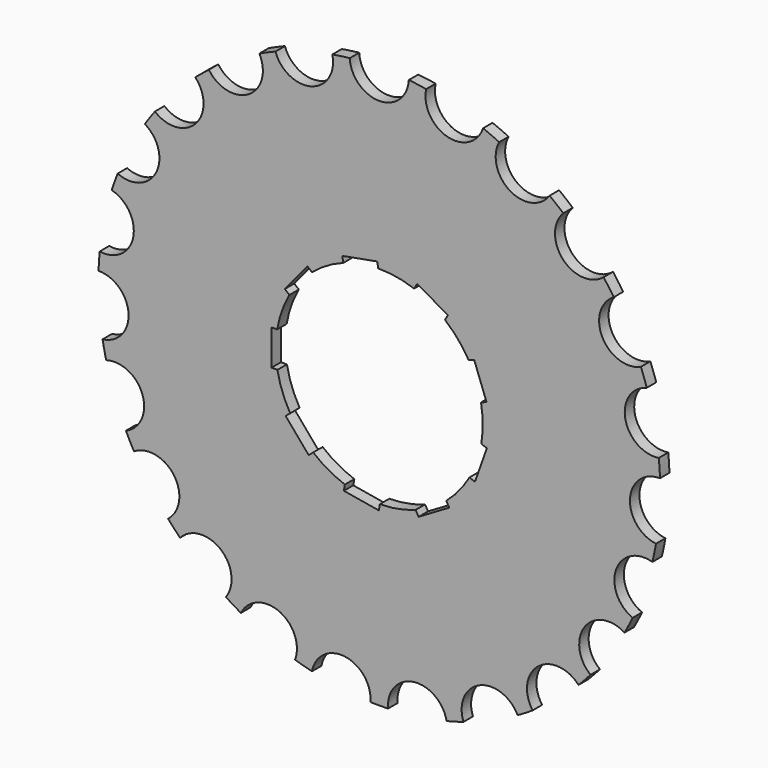
from build123d import *

# Parameters (mm, degrees)
F0_R            = 47.5
F0_R_2          = 17.5
F1_DEPTH        = 2
F3_DEPTH        = 2.001
F3_COPIES_COUNT = 23
F6_DEPTH        = 25
F6_COPIES_COUNT = 9


# Not quite as in the source:
# - a pattern or mirror of a feature is missing from the dataset's text; its kind, count and spacing are read off the source's solid


with BuildPart() as f1:
    # F0 (on Front) → F1 (new body)
    with BuildSketch(Plane.XZ):
        Circle(F0_R)
        Circle(F0_R_2, mode=Mode.SUBTRACT)
    extrude(amount=F1_DEPTH)

    # F2 (on face) → F3 (cut, through all)
    with BuildSketch(Plane.XZ.offset(2)):
        with BuildLine():
            ThreePointArc((4.9930699897, 47.2368421053), (0, 47.5), (-4.9930699897, 47.2368421053))
            ThreePointArc((-4.9930699897, 47.2368421053), (0, 42.5), (4.9930699897, 47.2368421053))
        make_face()
    f3 = extrude(amount=-F3_DEPTH, mode=Mode.SUBTRACT)

    # F3_copies: F3 ×23 about axis
    f3_copies_axis = Axis((0, 0, 0), (0, 1, 0))
    for i in range(1, F3_COPIES_COUNT):
        add(f3.rotate(f3_copies_axis, i * 360 / F3_COPIES_COUNT), mode=Mode.SUBTRACT)

    # F5 (on face) → F6 (cut)
    with BuildSketch(Plane.XZ.offset(2)):
        with BuildLine():
            Line((-6.2547624065, 17.3956841353), (-6.0736095937, 16.4122291753))
            ThreePointArc((-6.0736095937, 16.4122291753), (-3.1701742248, 17.2104618004), (-0.1728798335, 17.4991460524))
            Line((-0.1728798335, 17.4991460524), (-0.3540326464, 18.4826010124))
            Line((-0.3540326464, 18.4826010124), (-6.2547624065, 17.3956841353))
        make_face()
    f6 = extrude(amount=-F6_DEPTH, mode=Mode.SUBTRACT)

    # F6_copies: F6 ×9 about axis
    f6_copies_axis = Axis((0, 0, 0), (0, 1, 0))
    for i in range(1, F6_COPIES_COUNT):
        add(f6.rotate(f6_copies_axis, i * 360 / F6_COPIES_COUNT), mode=Mode.SUBTRACT)


solid = f1.part
